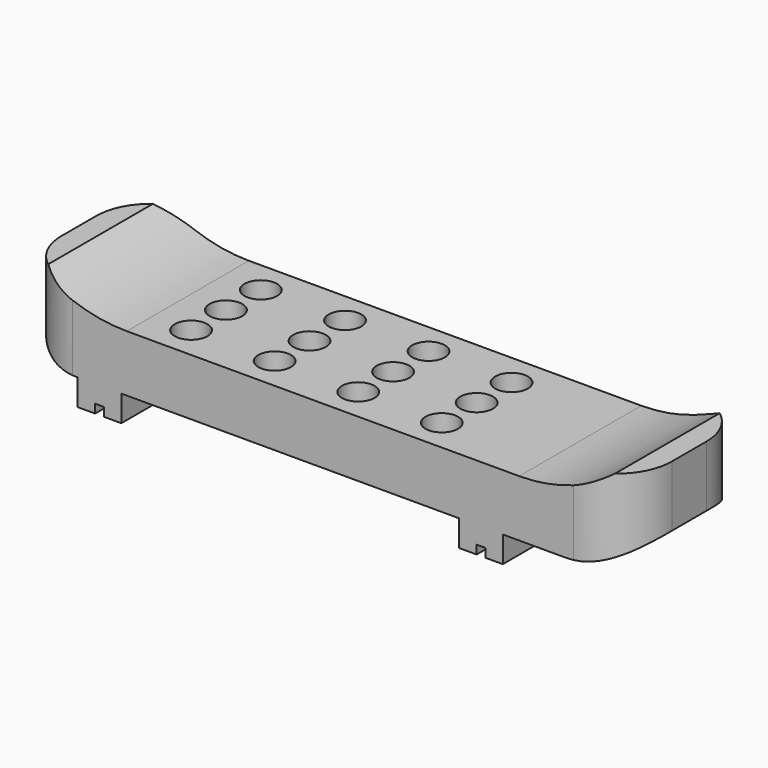
from build123d import *

# Parameters (mm, degrees)
F0_W          = 177.8
F0_H          = 31.75
F12_DEPTH     = 22.225
F1_W          = 2.54
F1_H          = 2.54
F2_DEPTH      = 22.225
F2_DEPTH_BACK = 22.225
F3_W          = 17.4625
F3_H          = 7.62
F3_W_2        = 98.425
F3_W_3        = 36.5125
F4_DEPTH      = 44.451
F6_DEPTH      = 44.451
F7_R          = 15.875
F9_D          = 9.525
F10_W         = 98.425
F10_H         = 44.45
F11_DEPTH     = 2.54


# Not quite as in the source:
# - a length typed as a fraction of an inch, garbled in the dataset ("3 / 203.2 mm" for 3/8 in), is restored


with BuildPart() as f12:
    # F0 (on Front) → F12 (new body, symmetric)
    with BuildSketch(Plane.XZ):
        Rectangle(F0_W, F0_H)
    extrude(amount=F12_DEPTH, both=True)

    # F1 (on Front) → F2 (cut, two sides)
    with BuildSketch(Plane.XZ) as f2_sk:
        with Locations((-65.0875, -14.605)):
            Rectangle(F1_W, F1_H)
        with Locations((46.0375, -14.605)):
            Rectangle(F1_W, F1_H)
    extrude(amount=F2_DEPTH, mode=Mode.SUBTRACT)
    extrude(f2_sk.sketch, amount=-F2_DEPTH_BACK, mode=Mode.SUBTRACT)

    # F3 (on face) → F4 (cut, through all)
    with BuildSketch(Plane.XZ.offset(22.225)):
        with Locations((-80.16875, -12.065)):
            Rectangle(F3_W, F3_H)
        with Locations((-9.525, -12.065)):
            Rectangle(F3_W_2, F3_H)
        with Locations((70.64375, -12.065)):
            Rectangle(F3_W_3, F3_H)
    extrude(amount=-F4_DEPTH, mode=Mode.SUBTRACT)

    # F5 (on face) → F6 (cut, through all)
    with BuildSketch(Plane.XZ.offset(22.225)):
        with BuildLine():
            Line((82.55, 15.875), (-82.55, 15.875))
            ThreePointArc((-82.55, 15.875), (-70.4091892663, 10.2010357789), (-57.15, 8.255))
            Line((-57.15, 8.255), (57.15, 8.255))
            ThreePointArc((57.15, 8.255), (70.4091892663, 10.2010357789), (82.55, 15.875))
        make_face()
        with BuildLine():
            ThreePointArc((-71.12, -8.255), (-80.5599536545, -6.6198702327), (-88.9, -1.905))
            Line((-88.9, -1.905), (-88.9, -8.255))
            Line((-88.9, -8.255), (-71.4375, -8.255))
            Line((-71.4375, -8.255), (-71.12, -8.255))
        make_face()
        with BuildLine():
            Line((88.9, -8.255), (88.9, -1.905))
            ThreePointArc((88.9, -1.905), (79.890231571, -6.6256947131), (69.85, -8.255))
            Line((69.85, -8.255), (88.9, -8.255))
        make_face()
    extrude(amount=-F6_DEPTH, mode=Mode.SUBTRACT)

    # F7
    f7_edges = [f12.edges().sort_by_distance(p)[0] for p in [
        (-88.9, -22.225, 6.985),
        (88.9, -22.225, 6.985),
        (88.9, 22.225, 6.985),
        (-88.9, 22.225, 6.985),
    ]]
    fillet(f7_edges, radius=F7_R)

    # F9 (through all)
    with Locations(Plane(origin=(0, 0, -8.255), x_dir=(1, 0, 0), z_dir=(0, 0, -1))):
        with Locations((-46.0375, 12.7), (-46.0375, 0), (-46.0375, -12.7), (26.9875, -12.7), (26.9875, 0), (26.9875, 12.7), (-21.6958333333, 12.7), (2.6458333333, 12.7), (2.6458333333, 0), (-21.6958333333, 0), (-21.6958333333, -12.924679948), (2.6458333333, -12.924679948)):
            Hole(F9_D / 2)

    # F10 (on face) → F11 (join)
    with BuildSketch(Plane(origin=(0, 0, -8.255), x_dir=(1, 0, 0), z_dir=(0, 0, -1))):
        with Locations((-9.525, 0)):
            Rectangle(F10_W, F10_H)
    extrude(amount=-F11_DEPTH)


solid = f12.part
